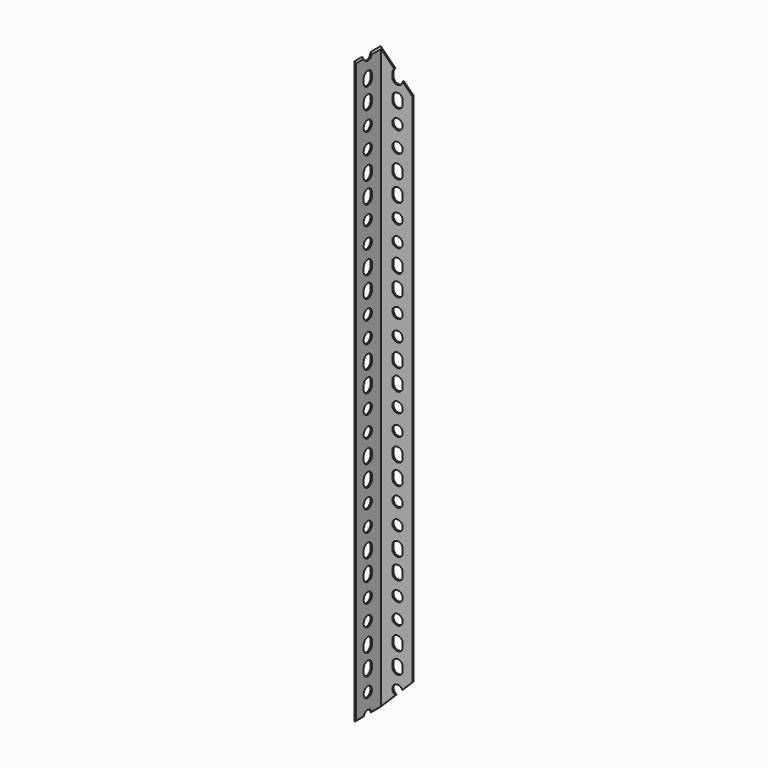
from build123d import *

# Parameters (mm, degrees)
F2_DEPTH = 533.4
F3_R     = 4.7625
F5_DEPTH = 1.3726
F4_R     = 4.7625
F6_DEPTH = 1.3726
F8_DEPTH = 30.1254


# Not quite as in the source:
# - a variable given as a bare number and used for a length is read in inches; the dataset says mm whatever the document's units were


with BuildPart() as f2:
    # F1 (on Top) → F2 (new body)
    with BuildSketch(Plane.XY):
        Polygon((-1.3716, 1.3716), (-1.3716, -28.7528), (0, -28.7528), (0, 0), (28.7528, 0), (28.7528, 1.3716), align=None)
    extrude(amount=F2_DEPTH)

    # F3 (on face) → F5 (cut, through all)
    with BuildSketch(Plane.XZ):
        with Locations((15.1384, 19.05)):
            Circle(F3_R)
        with Locations((15.1384, 0)):
            Circle(F3_R)
        with BuildLine():
            Line((19.9009, 36.5125), (19.9009, 39.6875))
            ThreePointArc((19.9009, 39.6875), (15.1384, 44.45), (10.3759, 39.6875))
            Line((10.3759, 39.6875), (10.3759, 36.5125))
            ThreePointArc((10.3759, 36.5125), (15.1384, 31.75), (19.9009, 36.5125))
        make_face()
        with BuildLine():
            Line((19.9009, 55.5625), (19.9009, 58.7375))
            ThreePointArc((19.9009, 58.7375), (15.1384, 63.5), (10.3759, 58.7375))
            Line((10.3759, 58.7375), (10.3759, 55.5625))
            ThreePointArc((10.3759, 55.5625), (15.1384, 50.8), (19.9009, 55.5625))
        make_face()
        with BuildLine():
            Line((19.9009, 131.7625), (19.9009, 134.9375))
            ThreePointArc((19.9009, 134.9375), (15.1384, 139.7), (10.3759, 134.9375))
            Line((10.3759, 134.9375), (10.3759, 131.7625))
            ThreePointArc((10.3759, 131.7625), (15.1384, 127), (19.9009, 131.7625))
        make_face()
        with Locations((15.1384, 95.25)):
            Circle(F3_R)
        with Locations((15.1384, 76.2)):
            Circle(F3_R)
        with BuildLine():
            Line((19.9009, 112.7125), (19.9009, 115.8875))
            ThreePointArc((19.9009, 115.8875), (15.1384, 120.65), (10.3759, 115.8875))
            Line((10.3759, 115.8875), (10.3759, 112.7125))
            ThreePointArc((10.3759, 112.7125), (15.1384, 107.95), (19.9009, 112.7125))
        make_face()
        with BuildLine():
            Line((19.9009, 207.9625), (19.9009, 211.1375))
            ThreePointArc((19.9009, 211.1375), (15.1384, 215.9), (10.3759, 211.1375))
            Line((10.3759, 211.1375), (10.3759, 207.9625))
            ThreePointArc((10.3759, 207.9625), (15.1384, 203.2), (19.9009, 207.9625))
        make_face()
        with Locations((15.1384, 171.45)):
            Circle(F3_R)
        with Locations((15.1384, 152.4)):
            Circle(F3_R)
        with BuildLine():
            Line((19.9009, 188.9125), (19.9009, 192.0875))
            ThreePointArc((19.9009, 192.0875), (15.1384, 196.85), (10.3759, 192.0875))
            Line((10.3759, 192.0875), (10.3759, 188.9125))
            ThreePointArc((10.3759, 188.9125), (15.1384, 184.15), (19.9009, 188.9125))
        make_face()
        with BuildLine():
            Line((19.9009, 284.1625), (19.9009, 287.3375))
            ThreePointArc((19.9009, 287.3375), (15.1384, 292.1), (10.3759, 287.3375))
            Line((10.3759, 287.3375), (10.3759, 284.1625))
            ThreePointArc((10.3759, 284.1625), (15.1384, 279.4), (19.9009, 284.1625))
        make_face()
        with Locations((15.1384, 247.65)):
            Circle(F3_R)
        with Locations((15.1384, 228.6)):
            Circle(F3_R)
        with BuildLine():
            Line((19.9009, 265.1125), (19.9009, 268.2875))
            ThreePointArc((19.9009, 268.2875), (15.1384, 273.05), (10.3759, 268.2875))
            Line((10.3759, 268.2875), (10.3759, 265.1125))
            ThreePointArc((10.3759, 265.1125), (15.1384, 260.35), (19.9009, 265.1125))
        make_face()
        with BuildLine():
            Line((19.9009, 360.3625), (19.9009, 363.5375))
            ThreePointArc((19.9009, 363.5375), (15.1384, 368.3), (10.3759, 363.5375))
            Line((10.3759, 363.5375), (10.3759, 360.3625))
            ThreePointArc((10.3759, 360.3625), (15.1384, 355.6), (19.9009, 360.3625))
        make_face()
        with Locations((15.1384, 323.85)):
            Circle(F3_R)
        with Locations((15.1384, 304.8)):
            Circle(F3_R)
        with BuildLine():
            Line((19.9009, 341.3125), (19.9009, 344.4875))
            ThreePointArc((19.9009, 344.4875), (15.1384, 349.25), (10.3759, 344.4875))
            Line((10.3759, 344.4875), (10.3759, 341.3125))
            ThreePointArc((10.3759, 341.3125), (15.1384, 336.55), (19.9009, 341.3125))
        make_face()
        with BuildLine():
            Line((19.9009, 436.5625), (19.9009, 439.7375))
            ThreePointArc((19.9009, 439.7375), (15.1384, 444.5), (10.3759, 439.7375))
            Line((10.3759, 439.7375), (10.3759, 436.5625))
            ThreePointArc((10.3759, 436.5625), (15.1384, 431.8), (19.9009, 436.5625))
        make_face()
        with Locations((15.1384, 400.05)):
            Circle(F3_R)
        with Locations((15.1384, 381)):
            Circle(F3_R)
        with BuildLine():
            Line((19.9009, 417.5125), (19.9009, 420.6875))
            ThreePointArc((19.9009, 420.6875), (15.1384, 425.45), (10.3759, 420.6875))
            Line((10.3759, 420.6875), (10.3759, 417.5125))
            ThreePointArc((10.3759, 417.5125), (15.1384, 412.75), (19.9009, 417.5125))
        make_face()
        with BuildLine():
            Line((19.9009, 512.7625), (19.9009, 515.9375))
            ThreePointArc((19.9009, 515.9375), (15.1384, 520.7), (10.3759, 515.9375))
            Line((10.3759, 515.9375), (10.3759, 512.7625))
            ThreePointArc((10.3759, 512.7625), (15.1384, 508), (19.9009, 512.7625))
        make_face()
        with Locations((15.1384, 476.25)):
            Circle(F3_R)
        with Locations((15.1384, 457.2)):
            Circle(F3_R)
        with BuildLine():
            Line((19.9009, 493.7125), (19.9009, 496.8875))
            ThreePointArc((19.9009, 496.8875), (15.1384, 501.65), (10.3759, 496.8875))
            Line((10.3759, 496.8875), (10.3759, 493.7125))
            ThreePointArc((10.3759, 493.7125), (15.1384, 488.95), (19.9009, 493.7125))
        make_face()
        with BuildLine():
            Line((19.9009, 588.9625), (19.9009, 592.1375))
            ThreePointArc((19.9009, 592.1375), (15.1384, 596.9), (10.3759, 592.1375))
            Line((10.3759, 592.1375), (10.3759, 588.9625))
            ThreePointArc((10.3759, 588.9625), (15.1384, 584.2), (19.9009, 588.9625))
        make_face()
        with Locations((15.1384, 552.45)):
            Circle(F3_R)
        with Locations((15.1384, 533.4)):
            Circle(F3_R)
        with BuildLine():
            Line((19.9009, 569.9125), (19.9009, 573.0875))
            ThreePointArc((19.9009, 573.0875), (15.1384, 577.85), (10.3759, 573.0875))
            Line((10.3759, 573.0875), (10.3759, 569.9125))
            ThreePointArc((10.3759, 569.9125), (15.1384, 565.15), (19.9009, 569.9125))
        make_face()
        with BuildLine():
            Line((19.9009, 665.1625), (19.9009, 668.3375))
            ThreePointArc((19.9009, 668.3375), (15.1384, 673.1), (10.3759, 668.3375))
            Line((10.3759, 668.3375), (10.3759, 665.1625))
            ThreePointArc((10.3759, 665.1625), (15.1384, 660.4), (19.9009, 665.1625))
        make_face()
        with Locations((15.1384, 628.65)):
            Circle(F3_R)
        with Locations((15.1384, 609.6)):
            Circle(F3_R)
        with BuildLine():
            Line((19.9009, 646.1125), (19.9009, 649.2875))
            ThreePointArc((19.9009, 649.2875), (15.1384, 654.05), (10.3759, 649.2875))
            Line((10.3759, 649.2875), (10.3759, 646.1125))
            ThreePointArc((10.3759, 646.1125), (15.1384, 641.35), (19.9009, 646.1125))
        make_face()
        with BuildLine():
            Line((19.9009, 741.3625), (19.9009, 744.5375))
            ThreePointArc((19.9009, 744.5375), (15.1384, 749.3), (10.3759, 744.5375))
            Line((10.3759, 744.5375), (10.3759, 741.3625))
            ThreePointArc((10.3759, 741.3625), (15.1384, 736.6), (19.9009, 741.3625))
        make_face()
        with Locations((15.1384, 704.85)):
            Circle(F3_R)
        with Locations((15.1384, 685.8)):
            Circle(F3_R)
        with BuildLine():
            Line((19.9009, 722.3125), (19.9009, 725.4875))
            ThreePointArc((19.9009, 725.4875), (15.1384, 730.25), (10.3759, 725.4875))
            Line((10.3759, 725.4875), (10.3759, 722.3125))
            ThreePointArc((10.3759, 722.3125), (15.1384, 717.55), (19.9009, 722.3125))
        make_face()
        with BuildLine():
            Line((19.9009, 817.5625), (19.9009, 820.7375))
            ThreePointArc((19.9009, 820.7375), (15.1384, 825.5), (10.3759, 820.7375))
            Line((10.3759, 820.7375), (10.3759, 817.5625))
            ThreePointArc((10.3759, 817.5625), (15.1384, 812.8), (19.9009, 817.5625))
        make_face()
        with Locations((15.1384, 781.05)):
            Circle(F3_R)
        with Locations((15.1384, 762)):
            Circle(F3_R)
        with BuildLine():
            Line((19.9009, 798.5125), (19.9009, 801.6875))
            ThreePointArc((19.9009, 801.6875), (15.1384, 806.45), (10.3759, 801.6875))
            Line((10.3759, 801.6875), (10.3759, 798.5125))
            ThreePointArc((10.3759, 798.5125), (15.1384, 793.75), (19.9009, 798.5125))
        make_face()
        with BuildLine():
            Line((19.9009, 893.7625), (19.9009, 896.9375))
            ThreePointArc((19.9009, 896.9375), (15.1384, 901.7), (10.3759, 896.9375))
            Line((10.3759, 896.9375), (10.3759, 893.7625))
            ThreePointArc((10.3759, 893.7625), (15.1384, 889), (19.9009, 893.7625))
        make_face()
        with Locations((15.1384, 857.25)):
            Circle(F3_R)
        with Locations((15.1384, 838.2)):
            Circle(F3_R)
        with BuildLine():
            Line((19.9009, 874.7125), (19.9009, 877.8875))
            ThreePointArc((19.9009, 877.8875), (15.1384, 882.65), (10.3759, 877.8875))
            Line((10.3759, 877.8875), (10.3759, 874.7125))
            ThreePointArc((10.3759, 874.7125), (15.1384, 869.95), (19.9009, 874.7125))
        make_face()
        with BuildLine():
            Line((19.9009, 969.9625), (19.9009, 973.1375))
            ThreePointArc((19.9009, 973.1375), (15.1384, 977.9), (10.3759, 973.1375))
            Line((10.3759, 973.1375), (10.3759, 969.9625))
            ThreePointArc((10.3759, 969.9625), (15.1384, 965.2), (19.9009, 969.9625))
        make_face()
        with Locations((15.1384, 933.45)):
            Circle(F3_R)
        with Locations((15.1384, 914.4)):
            Circle(F3_R)
        with BuildLine():
            Line((19.9009, 950.9125), (19.9009, 954.0875))
            ThreePointArc((19.9009, 954.0875), (15.1384, 958.85), (10.3759, 954.0875))
            Line((10.3759, 954.0875), (10.3759, 950.9125))
            ThreePointArc((10.3759, 950.9125), (15.1384, 946.15), (19.9009, 950.9125))
        make_face()
        with BuildLine():
            Line((19.9009, 1046.1625), (19.9009, 1049.3375))
            ThreePointArc((19.9009, 1049.3375), (15.1384, 1054.1), (10.3759, 1049.3375))
            Line((10.3759, 1049.3375), (10.3759, 1046.1625))
            ThreePointArc((10.3759, 1046.1625), (15.1384, 1041.4), (19.9009, 1046.1625))
        make_face()
        with Locations((15.1384, 1009.65)):
            Circle(F3_R)
        with Locations((15.1384, 990.6)):
            Circle(F3_R)
        with BuildLine():
            Line((19.9009, 1027.1125), (19.9009, 1030.2875))
            ThreePointArc((19.9009, 1030.2875), (15.1384, 1035.05), (10.3759, 1030.2875))
            Line((10.3759, 1030.2875), (10.3759, 1027.1125))
            ThreePointArc((10.3759, 1027.1125), (15.1384, 1022.35), (19.9009, 1027.1125))
        make_face()
        with BuildLine():
            Line((19.9009, 1122.3625), (19.9009, 1125.5375))
            ThreePointArc((19.9009, 1125.5375), (15.1384, 1130.3), (10.3759, 1125.5375))
            Line((10.3759, 1125.5375), (10.3759, 1122.3625))
            ThreePointArc((10.3759, 1122.3625), (15.1384, 1117.6), (19.9009, 1122.3625))
        make_face()
        with Locations((15.1384, 1085.85)):
            Circle(F3_R)
        with Locations((15.1384, 1066.8)):
            Circle(F3_R)
        with BuildLine():
            Line((19.9009, 1103.3125), (19.9009, 1106.4875))
            ThreePointArc((19.9009, 1106.4875), (15.1384, 1111.25), (10.3759, 1106.4875))
            Line((10.3759, 1106.4875), (10.3759, 1103.3125))
            ThreePointArc((10.3759, 1103.3125), (15.1384, 1098.55), (19.9009, 1103.3125))
        make_face()
        with BuildLine():
            Line((19.9009, 1198.5625), (19.9009, 1201.7375))
            ThreePointArc((19.9009, 1201.7375), (15.1384, 1206.5), (10.3759, 1201.7375))
            Line((10.3759, 1201.7375), (10.3759, 1198.5625))
            ThreePointArc((10.3759, 1198.5625), (15.1384, 1193.8), (19.9009, 1198.5625))
        make_face()
        with Locations((15.1384, 1162.05)):
            Circle(F3_R)
        with Locations((15.1384, 1143)):
            Circle(F3_R)
        with BuildLine():
            Line((19.9009, 1179.5125), (19.9009, 1182.6875))
            ThreePointArc((19.9009, 1182.6875), (15.1384, 1187.45), (10.3759, 1182.6875))
            Line((10.3759, 1182.6875), (10.3759, 1179.5125))
            ThreePointArc((10.3759, 1179.5125), (15.1384, 1174.75), (19.9009, 1179.5125))
        make_face()
        with BuildLine():
            Line((19.9009, 1274.7625), (19.9009, 1277.9375))
            ThreePointArc((19.9009, 1277.9375), (15.1384, 1282.7), (10.3759, 1277.9375))
            Line((10.3759, 1277.9375), (10.3759, 1274.7625))
            ThreePointArc((10.3759, 1274.7625), (15.1384, 1270), (19.9009, 1274.7625))
        make_face()
        with Locations((15.1384, 1238.25)):
            Circle(F3_R)
        with Locations((15.1384, 1219.2)):
            Circle(F3_R)
        with BuildLine():
            Line((19.9009, 1255.7125), (19.9009, 1258.8875))
            ThreePointArc((19.9009, 1258.8875), (15.1384, 1263.65), (10.3759, 1258.8875))
            Line((10.3759, 1258.8875), (10.3759, 1255.7125))
            ThreePointArc((10.3759, 1255.7125), (15.1384, 1250.95), (19.9009, 1255.7125))
        make_face()
        with BuildLine():
            Line((19.9009, 1350.9625), (19.9009, 1354.1375))
            ThreePointArc((19.9009, 1354.1375), (15.1384, 1358.9), (10.3759, 1354.1375))
            Line((10.3759, 1354.1375), (10.3759, 1350.9625))
            ThreePointArc((10.3759, 1350.9625), (15.1384, 1346.2), (19.9009, 1350.9625))
        make_face()
        with Locations((15.1384, 1314.45)):
            Circle(F3_R)
        with Locations((15.1384, 1295.4)):
            Circle(F3_R)
        with BuildLine():
            Line((19.9009, 1331.9125), (19.9009, 1335.0875))
            ThreePointArc((19.9009, 1335.0875), (15.1384, 1339.85), (10.3759, 1335.0875))
            Line((10.3759, 1335.0875), (10.3759, 1331.9125))
            ThreePointArc((10.3759, 1331.9125), (15.1384, 1327.15), (19.9009, 1331.9125))
        make_face()
        with BuildLine():
            Line((19.9009, 1427.1625), (19.9009, 1430.3375))
            ThreePointArc((19.9009, 1430.3375), (15.1384, 1435.1), (10.3759, 1430.3375))
            Line((10.3759, 1430.3375), (10.3759, 1427.1625))
            ThreePointArc((10.3759, 1427.1625), (15.1384, 1422.4), (19.9009, 1427.1625))
        make_face()
        with Locations((15.1384, 1390.65)):
            Circle(F3_R)
        with Locations((15.1384, 1371.6)):
            Circle(F3_R)
        with BuildLine():
            Line((19.9009, 1408.1125), (19.9009, 1411.2875))
            ThreePointArc((19.9009, 1411.2875), (15.1384, 1416.05), (10.3759, 1411.2875))
            Line((10.3759, 1411.2875), (10.3759, 1408.1125))
            ThreePointArc((10.3759, 1408.1125), (15.1384, 1403.35), (19.9009, 1408.1125))
        make_face()
        with BuildLine():
            Line((19.9009, 1503.3625), (19.9009, 1506.5375))
            ThreePointArc((19.9009, 1506.5375), (15.1384, 1511.3), (10.3759, 1506.5375))
            Line((10.3759, 1506.5375), (10.3759, 1503.3625))
            ThreePointArc((10.3759, 1503.3625), (15.1384, 1498.6), (19.9009, 1503.3625))
        make_face()
        with Locations((15.1384, 1466.85)):
            Circle(F3_R)
        with Locations((15.1384, 1447.8)):
            Circle(F3_R)
        with BuildLine():
            Line((19.9009, 1484.3125), (19.9009, 1487.4875))
            ThreePointArc((19.9009, 1487.4875), (15.1384, 1492.25), (10.3759, 1487.4875))
            Line((10.3759, 1487.4875), (10.3759, 1484.3125))
            ThreePointArc((10.3759, 1484.3125), (15.1384, 1479.55), (19.9009, 1484.3125))
        make_face()
        with BuildLine():
            Line((19.9009, 1579.5625), (19.9009, 1582.7375))
            ThreePointArc((19.9009, 1582.7375), (15.1384, 1587.5), (10.3759, 1582.7375))
            Line((10.3759, 1582.7375), (10.3759, 1579.5625))
            ThreePointArc((10.3759, 1579.5625), (15.1384, 1574.8), (19.9009, 1579.5625))
        make_face()
        with Locations((15.1384, 1543.05)):
            Circle(F3_R)
        with Locations((15.1384, 1524)):
            Circle(F3_R)
        with BuildLine():
            Line((19.9009, 1560.5125), (19.9009, 1563.6875))
            ThreePointArc((19.9009, 1563.6875), (15.1384, 1568.45), (10.3759, 1563.6875))
            Line((10.3759, 1563.6875), (10.3759, 1560.5125))
            ThreePointArc((10.3759, 1560.5125), (15.1384, 1555.75), (19.9009, 1560.5125))
        make_face()
        with BuildLine():
            Line((19.9009, 1655.7625), (19.9009, 1658.9375))
            ThreePointArc((19.9009, 1658.9375), (15.1384, 1663.7), (10.3759, 1658.9375))
            Line((10.3759, 1658.9375), (10.3759, 1655.7625))
            ThreePointArc((10.3759, 1655.7625), (15.1384, 1651), (19.9009, 1655.7625))
        make_face()
        with Locations((15.1384, 1619.25)):
            Circle(F3_R)
        with Locations((15.1384, 1600.2)):
            Circle(F3_R)
        with BuildLine():
            Line((19.9009, 1636.7125), (19.9009, 1639.8875))
            ThreePointArc((19.9009, 1639.8875), (15.1384, 1644.65), (10.3759, 1639.8875))
            Line((10.3759, 1639.8875), (10.3759, 1636.7125))
            ThreePointArc((10.3759, 1636.7125), (15.1384, 1631.95), (19.9009, 1636.7125))
        make_face()
        with BuildLine():
            Line((19.9009, 1731.9625), (19.9009, 1735.1375))
            ThreePointArc((19.9009, 1735.1375), (15.1384, 1739.9), (10.3759, 1735.1375))
            Line((10.3759, 1735.1375), (10.3759, 1731.9625))
            ThreePointArc((10.3759, 1731.9625), (15.1384, 1727.2), (19.9009, 1731.9625))
        make_face()
        with Locations((15.1384, 1695.45)):
            Circle(F3_R)
        with Locations((15.1384, 1676.4)):
            Circle(F3_R)
        with BuildLine():
            Line((19.9009, 1712.9125), (19.9009, 1716.0875))
            ThreePointArc((19.9009, 1716.0875), (15.1384, 1720.85), (10.3759, 1716.0875))
            Line((10.3759, 1716.0875), (10.3759, 1712.9125))
            ThreePointArc((10.3759, 1712.9125), (15.1384, 1708.15), (19.9009, 1712.9125))
        make_face()
        with BuildLine():
            Line((19.9009, 1808.1625), (19.9009, 1811.3375))
            ThreePointArc((19.9009, 1811.3375), (15.1384, 1816.1), (10.3759, 1811.3375))
            Line((10.3759, 1811.3375), (10.3759, 1808.1625))
            ThreePointArc((10.3759, 1808.1625), (15.1384, 1803.4), (19.9009, 1808.1625))
        make_face()
        with Locations((15.1384, 1771.65)):
            Circle(F3_R)
        with Locations((15.1384, 1752.6)):
            Circle(F3_R)
        with BuildLine():
            Line((19.9009, 1789.1125), (19.9009, 1792.2875))
            ThreePointArc((19.9009, 1792.2875), (15.1384, 1797.05), (10.3759, 1792.2875))
            Line((10.3759, 1792.2875), (10.3759, 1789.1125))
            ThreePointArc((10.3759, 1789.1125), (15.1384, 1784.35), (19.9009, 1789.1125))
        make_face()
    extrude(amount=-F5_DEPTH, mode=Mode.SUBTRACT)

    # F4 (on face) → F6 (cut, through all)
    with BuildSketch(Plane.YZ):
        with Locations((-15.1384, 19.05)):
            Circle(F4_R)
        with Locations((-15.1384, 0)):
            Circle(F4_R)
        with BuildLine():
            Line((-10.3759, 36.5125), (-10.3759, 39.6875))
            ThreePointArc((-10.3759, 39.6875), (-15.1384, 44.45), (-19.9009, 39.6875))
            Line((-19.9009, 39.6875), (-19.9009, 36.5125))
            ThreePointArc((-19.9009, 36.5125), (-15.1384, 31.75), (-10.3759, 36.5125))
        make_face()
        with BuildLine():
            Line((-10.3759, 55.5625), (-10.3759, 58.7375))
            ThreePointArc((-10.3759, 58.7375), (-15.1384, 63.5), (-19.9009, 58.7375))
            Line((-19.9009, 58.7375), (-19.9009, 55.5625))
            ThreePointArc((-19.9009, 55.5625), (-15.1384, 50.8), (-10.3759, 55.5625))
        make_face()
        with BuildLine():
            Line((-10.3759, 131.7625), (-10.3759, 134.9375))
            ThreePointArc((-10.3759, 134.9375), (-15.1384, 139.7), (-19.9009, 134.9375))
            Line((-19.9009, 134.9375), (-19.9009, 131.7625))
            ThreePointArc((-19.9009, 131.7625), (-15.1384, 127), (-10.3759, 131.7625))
        make_face()
        with Locations((-15.1384, 95.25)):
            Circle(F4_R)
        with Locations((-15.1384, 76.2)):
            Circle(F4_R)
        with BuildLine():
            Line((-10.3759, 112.7125), (-10.3759, 115.8875))
            ThreePointArc((-10.3759, 115.8875), (-15.1384, 120.65), (-19.9009, 115.8875))
            Line((-19.9009, 115.8875), (-19.9009, 112.7125))
            ThreePointArc((-19.9009, 112.7125), (-15.1384, 107.95), (-10.3759, 112.7125))
        make_face()
        with BuildLine():
            Line((-10.3759, 207.9625), (-10.3759, 211.1375))
            ThreePointArc((-10.3759, 211.1375), (-15.1384, 215.9), (-19.9009, 211.1375))
            Line((-19.9009, 211.1375), (-19.9009, 207.9625))
            ThreePointArc((-19.9009, 207.9625), (-15.1384, 203.2), (-10.3759, 207.9625))
        make_face()
        with Locations((-15.1384, 171.45)):
            Circle(F4_R)
        with Locations((-15.1384, 152.4)):
            Circle(F4_R)
        with BuildLine():
            Line((-10.3759, 188.9125), (-10.3759, 192.0875))
            ThreePointArc((-10.3759, 192.0875), (-15.1384, 196.85), (-19.9009, 192.0875))
            Line((-19.9009, 192.0875), (-19.9009, 188.9125))
            ThreePointArc((-19.9009, 188.9125), (-15.1384, 184.15), (-10.3759, 188.9125))
        make_face()
        with BuildLine():
            Line((-10.3759, 284.1625), (-10.3759, 287.3375))
            ThreePointArc((-10.3759, 287.3375), (-15.1384, 292.1), (-19.9009, 287.3375))
            Line((-19.9009, 287.3375), (-19.9009, 284.1625))
            ThreePointArc((-19.9009, 284.1625), (-15.1384, 279.4), (-10.3759, 284.1625))
        make_face()
        with Locations((-15.1384, 247.65)):
            Circle(F4_R)
        with Locations((-15.1384, 228.6)):
            Circle(F4_R)
        with BuildLine():
            Line((-10.3759, 265.1125), (-10.3759, 268.2875))
            ThreePointArc((-10.3759, 268.2875), (-15.1384, 273.05), (-19.9009, 268.2875))
            Line((-19.9009, 268.2875), (-19.9009, 265.1125))
            ThreePointArc((-19.9009, 265.1125), (-15.1384, 260.35), (-10.3759, 265.1125))
        make_face()
        with BuildLine():
            Line((-10.3759, 360.3625), (-10.3759, 363.5375))
            ThreePointArc((-10.3759, 363.5375), (-15.1384, 368.3), (-19.9009, 363.5375))
            Line((-19.9009, 363.5375), (-19.9009, 360.3625))
            ThreePointArc((-19.9009, 360.3625), (-15.1384, 355.6), (-10.3759, 360.3625))
        make_face()
        with Locations((-15.1384, 323.85)):
            Circle(F4_R)
        with Locations((-15.1384, 304.8)):
            Circle(F4_R)
        with BuildLine():
            Line((-10.3759, 341.3125), (-10.3759, 344.4875))
            ThreePointArc((-10.3759, 344.4875), (-15.1384, 349.25), (-19.9009, 344.4875))
            Line((-19.9009, 344.4875), (-19.9009, 341.3125))
            ThreePointArc((-19.9009, 341.3125), (-15.1384, 336.55), (-10.3759, 341.3125))
        make_face()
        with BuildLine():
            Line((-10.3759, 436.5625), (-10.3759, 439.7375))
            ThreePointArc((-10.3759, 439.7375), (-15.1384, 444.5), (-19.9009, 439.7375))
            Line((-19.9009, 439.7375), (-19.9009, 436.5625))
            ThreePointArc((-19.9009, 436.5625), (-15.1384, 431.8), (-10.3759, 436.5625))
        make_face()
        with Locations((-15.1384, 400.05)):
            Circle(F4_R)
        with Locations((-15.1384, 381)):
            Circle(F4_R)
        with BuildLine():
            Line((-10.3759, 417.5125), (-10.3759, 420.6875))
            ThreePointArc((-10.3759, 420.6875), (-15.1384, 425.45), (-19.9009, 420.6875))
            Line((-19.9009, 420.6875), (-19.9009, 417.5125))
            ThreePointArc((-19.9009, 417.5125), (-15.1384, 412.75), (-10.3759, 417.5125))
        make_face()
        with BuildLine():
            Line((-10.3759, 512.7625), (-10.3759, 515.9375))
            ThreePointArc((-10.3759, 515.9375), (-15.1384, 520.7), (-19.9009, 515.9375))
            Line((-19.9009, 515.9375), (-19.9009, 512.7625))
            ThreePointArc((-19.9009, 512.7625), (-15.1384, 508), (-10.3759, 512.7625))
        make_face()
        with Locations((-15.1384, 476.25)):
            Circle(F4_R)
        with Locations((-15.1384, 457.2)):
            Circle(F4_R)
        with BuildLine():
            Line((-10.3759, 493.7125), (-10.3759, 496.8875))
            ThreePointArc((-10.3759, 496.8875), (-15.1384, 501.65), (-19.9009, 496.8875))
            Line((-19.9009, 496.8875), (-19.9009, 493.7125))
            ThreePointArc((-19.9009, 493.7125), (-15.1384, 488.95), (-10.3759, 493.7125))
        make_face()
        with BuildLine():
            Line((-10.3759, 588.9625), (-10.3759, 592.1375))
            ThreePointArc((-10.3759, 592.1375), (-15.1384, 596.9), (-19.9009, 592.1375))
            Line((-19.9009, 592.1375), (-19.9009, 588.9625))
            ThreePointArc((-19.9009, 588.9625), (-15.1384, 584.2), (-10.3759, 588.9625))
        make_face()
        with Locations((-15.1384, 552.45)):
            Circle(F4_R)
        with Locations((-15.1384, 533.4)):
            Circle(F4_R)
        with BuildLine():
            Line((-10.3759, 569.9125), (-10.3759, 573.0875))
            ThreePointArc((-10.3759, 573.0875), (-15.1384, 577.85), (-19.9009, 573.0875))
            Line((-19.9009, 573.0875), (-19.9009, 569.9125))
            ThreePointArc((-19.9009, 569.9125), (-15.1384, 565.15), (-10.3759, 569.9125))
        make_face()
        with BuildLine():
            Line((-10.3759, 665.1625), (-10.3759, 668.3375))
            ThreePointArc((-10.3759, 668.3375), (-15.1384, 673.1), (-19.9009, 668.3375))
            Line((-19.9009, 668.3375), (-19.9009, 665.1625))
            ThreePointArc((-19.9009, 665.1625), (-15.1384, 660.4), (-10.3759, 665.1625))
        make_face()
        with Locations((-15.1384, 628.65)):
            Circle(F4_R)
        with Locations((-15.1384, 609.6)):
            Circle(F4_R)
        with BuildLine():
            Line((-10.3759, 646.1125), (-10.3759, 649.2875))
            ThreePointArc((-10.3759, 649.2875), (-15.1384, 654.05), (-19.9009, 649.2875))
            Line((-19.9009, 649.2875), (-19.9009, 646.1125))
            ThreePointArc((-19.9009, 646.1125), (-15.1384, 641.35), (-10.3759, 646.1125))
        make_face()
        with BuildLine():
            Line((-10.3759, 741.3625), (-10.3759, 744.5375))
            ThreePointArc((-10.3759, 744.5375), (-15.1384, 749.3), (-19.9009, 744.5375))
            Line((-19.9009, 744.5375), (-19.9009, 741.3625))
            ThreePointArc((-19.9009, 741.3625), (-15.1384, 736.6), (-10.3759, 741.3625))
        make_face()
        with Locations((-15.1384, 704.85)):
            Circle(F4_R)
        with Locations((-15.1384, 685.8)):
            Circle(F4_R)
        with BuildLine():
            Line((-10.3759, 722.3125), (-10.3759, 725.4875))
            ThreePointArc((-10.3759, 725.4875), (-15.1384, 730.25), (-19.9009, 725.4875))
            Line((-19.9009, 725.4875), (-19.9009, 722.3125))
            ThreePointArc((-19.9009, 722.3125), (-15.1384, 717.55), (-10.3759, 722.3125))
        make_face()
        with BuildLine():
            Line((-10.3759, 817.5625), (-10.3759, 820.7375))
            ThreePointArc((-10.3759, 820.7375), (-15.1384, 825.5), (-19.9009, 820.7375))
            Line((-19.9009, 820.7375), (-19.9009, 817.5625))
            ThreePointArc((-19.9009, 817.5625), (-15.1384, 812.8), (-10.3759, 817.5625))
        make_face()
        with Locations((-15.1384, 781.05)):
            Circle(F4_R)
        with Locations((-15.1384, 762)):
            Circle(F4_R)
        with BuildLine():
            Line((-10.3759, 798.5125), (-10.3759, 801.6875))
            ThreePointArc((-10.3759, 801.6875), (-15.1384, 806.45), (-19.9009, 801.6875))
            Line((-19.9009, 801.6875), (-19.9009, 798.5125))
            ThreePointArc((-19.9009, 798.5125), (-15.1384, 793.75), (-10.3759, 798.5125))
        make_face()
        with BuildLine():
            Line((-10.3759, 893.7625), (-10.3759, 896.9375))
            ThreePointArc((-10.3759, 896.9375), (-15.1384, 901.7), (-19.9009, 896.9375))
            Line((-19.9009, 896.9375), (-19.9009, 893.7625))
            ThreePointArc((-19.9009, 893.7625), (-15.1384, 889), (-10.3759, 893.7625))
        make_face()
        with Locations((-15.1384, 857.25)):
            Circle(F4_R)
        with Locations((-15.1384, 838.2)):
            Circle(F4_R)
        with BuildLine():
            Line((-10.3759, 874.7125), (-10.3759, 877.8875))
            ThreePointArc((-10.3759, 877.8875), (-15.1384, 882.65), (-19.9009, 877.8875))
            Line((-19.9009, 877.8875), (-19.9009, 874.7125))
            ThreePointArc((-19.9009, 874.7125), (-15.1384, 869.95), (-10.3759, 874.7125))
        make_face()
        with BuildLine():
            Line((-10.3759, 969.9625), (-10.3759, 973.1375))
            ThreePointArc((-10.3759, 973.1375), (-15.1384, 977.9), (-19.9009, 973.1375))
            Line((-19.9009, 973.1375), (-19.9009, 969.9625))
            ThreePointArc((-19.9009, 969.9625), (-15.1384, 965.2), (-10.3759, 969.9625))
        make_face()
        with Locations((-15.1384, 933.45)):
            Circle(F4_R)
        with Locations((-15.1384, 914.4)):
            Circle(F4_R)
        with BuildLine():
            Line((-10.3759, 950.9125), (-10.3759, 954.0875))
            ThreePointArc((-10.3759, 954.0875), (-15.1384, 958.85), (-19.9009, 954.0875))
            Line((-19.9009, 954.0875), (-19.9009, 950.9125))
            ThreePointArc((-19.9009, 950.9125), (-15.1384, 946.15), (-10.3759, 950.9125))
        make_face()
        with BuildLine():
            Line((-10.3759, 1046.1625), (-10.3759, 1049.3375))
            ThreePointArc((-10.3759, 1049.3375), (-15.1384, 1054.1), (-19.9009, 1049.3375))
            Line((-19.9009, 1049.3375), (-19.9009, 1046.1625))
            ThreePointArc((-19.9009, 1046.1625), (-15.1384, 1041.4), (-10.3759, 1046.1625))
        make_face()
        with Locations((-15.1384, 1009.65)):
            Circle(F4_R)
        with Locations((-15.1384, 990.6)):
            Circle(F4_R)
        with BuildLine():
            Line((-10.3759, 1027.1125), (-10.3759, 1030.2875))
            ThreePointArc((-10.3759, 1030.2875), (-15.1384, 1035.05), (-19.9009, 1030.2875))
            Line((-19.9009, 1030.2875), (-19.9009, 1027.1125))
            ThreePointArc((-19.9009, 1027.1125), (-15.1384, 1022.35), (-10.3759, 1027.1125))
        make_face()
        with BuildLine():
            Line((-10.3759, 1122.3625), (-10.3759, 1125.5375))
            ThreePointArc((-10.3759, 1125.5375), (-15.1384, 1130.3), (-19.9009, 1125.5375))
            Line((-19.9009, 1125.5375), (-19.9009, 1122.3625))
            ThreePointArc((-19.9009, 1122.3625), (-15.1384, 1117.6), (-10.3759, 1122.3625))
        make_face()
        with Locations((-15.1384, 1085.85)):
            Circle(F4_R)
        with Locations((-15.1384, 1066.8)):
            Circle(F4_R)
        with BuildLine():
            Line((-10.3759, 1103.3125), (-10.3759, 1106.4875))
            ThreePointArc((-10.3759, 1106.4875), (-15.1384, 1111.25), (-19.9009, 1106.4875))
            Line((-19.9009, 1106.4875), (-19.9009, 1103.3125))
            ThreePointArc((-19.9009, 1103.3125), (-15.1384, 1098.55), (-10.3759, 1103.3125))
        make_face()
        with BuildLine():
            Line((-10.3759, 1198.5625), (-10.3759, 1201.7375))
            ThreePointArc((-10.3759, 1201.7375), (-15.1384, 1206.5), (-19.9009, 1201.7375))
            Line((-19.9009, 1201.7375), (-19.9009, 1198.5625))
            ThreePointArc((-19.9009, 1198.5625), (-15.1384, 1193.8), (-10.3759, 1198.5625))
        make_face()
        with Locations((-15.1384, 1162.05)):
            Circle(F4_R)
        with Locations((-15.1384, 1143)):
            Circle(F4_R)
        with BuildLine():
            Line((-10.3759, 1179.5125), (-10.3759, 1182.6875))
            ThreePointArc((-10.3759, 1182.6875), (-15.1384, 1187.45), (-19.9009, 1182.6875))
            Line((-19.9009, 1182.6875), (-19.9009, 1179.5125))
            ThreePointArc((-19.9009, 1179.5125), (-15.1384, 1174.75), (-10.3759, 1179.5125))
        make_face()
        with BuildLine():
            Line((-10.3759, 1274.7625), (-10.3759, 1277.9375))
            ThreePointArc((-10.3759, 1277.9375), (-15.1384, 1282.7), (-19.9009, 1277.9375))
            Line((-19.9009, 1277.9375), (-19.9009, 1274.7625))
            ThreePointArc((-19.9009, 1274.7625), (-15.1384, 1270), (-10.3759, 1274.7625))
        make_face()
        with Locations((-15.1384, 1238.25)):
            Circle(F4_R)
        with Locations((-15.1384, 1219.2)):
            Circle(F4_R)
        with BuildLine():
            Line((-10.3759, 1255.7125), (-10.3759, 1258.8875))
            ThreePointArc((-10.3759, 1258.8875), (-15.1384, 1263.65), (-19.9009, 1258.8875))
            Line((-19.9009, 1258.8875), (-19.9009, 1255.7125))
            ThreePointArc((-19.9009, 1255.7125), (-15.1384, 1250.95), (-10.3759, 1255.7125))
        make_face()
        with BuildLine():
            Line((-10.3759, 1350.9625), (-10.3759, 1354.1375))
            ThreePointArc((-10.3759, 1354.1375), (-15.1384, 1358.9), (-19.9009, 1354.1375))
            Line((-19.9009, 1354.1375), (-19.9009, 1350.9625))
            ThreePointArc((-19.9009, 1350.9625), (-15.1384, 1346.2), (-10.3759, 1350.9625))
        make_face()
        with Locations((-15.1384, 1314.45)):
            Circle(F4_R)
        with Locations((-15.1384, 1295.4)):
            Circle(F4_R)
        with BuildLine():
            Line((-10.3759, 1331.9125), (-10.3759, 1335.0875))
            ThreePointArc((-10.3759, 1335.0875), (-15.1384, 1339.85), (-19.9009, 1335.0875))
            Line((-19.9009, 1335.0875), (-19.9009, 1331.9125))
            ThreePointArc((-19.9009, 1331.9125), (-15.1384, 1327.15), (-10.3759, 1331.9125))
        make_face()
        with BuildLine():
            Line((-10.3759, 1427.1625), (-10.3759, 1430.3375))
            ThreePointArc((-10.3759, 1430.3375), (-15.1384, 1435.1), (-19.9009, 1430.3375))
            Line((-19.9009, 1430.3375), (-19.9009, 1427.1625))
            ThreePointArc((-19.9009, 1427.1625), (-15.1384, 1422.4), (-10.3759, 1427.1625))
        make_face()
        with Locations((-15.1384, 1390.65)):
            Circle(F4_R)
        with Locations((-15.1384, 1371.6)):
            Circle(F4_R)
        with BuildLine():
            Line((-10.3759, 1408.1125), (-10.3759, 1411.2875))
            ThreePointArc((-10.3759, 1411.2875), (-15.1384, 1416.05), (-19.9009, 1411.2875))
            Line((-19.9009, 1411.2875), (-19.9009, 1408.1125))
            ThreePointArc((-19.9009, 1408.1125), (-15.1384, 1403.35), (-10.3759, 1408.1125))
        make_face()
        with BuildLine():
            Line((-10.3759, 1503.3625), (-10.3759, 1506.5375))
            ThreePointArc((-10.3759, 1506.5375), (-15.1384, 1511.3), (-19.9009, 1506.5375))
            Line((-19.9009, 1506.5375), (-19.9009, 1503.3625))
            ThreePointArc((-19.9009, 1503.3625), (-15.1384, 1498.6), (-10.3759, 1503.3625))
        make_face()
        with Locations((-15.1384, 1466.85)):
            Circle(F4_R)
        with Locations((-15.1384, 1447.8)):
            Circle(F4_R)
        with BuildLine():
            Line((-10.3759, 1484.3125), (-10.3759, 1487.4875))
            ThreePointArc((-10.3759, 1487.4875), (-15.1384, 1492.25), (-19.9009, 1487.4875))
            Line((-19.9009, 1487.4875), (-19.9009, 1484.3125))
            ThreePointArc((-19.9009, 1484.3125), (-15.1384, 1479.55), (-10.3759, 1484.3125))
        make_face()
        with BuildLine():
            Line((-10.3759, 1579.5625), (-10.3759, 1582.7375))
            ThreePointArc((-10.3759, 1582.7375), (-15.1384, 1587.5), (-19.9009, 1582.7375))
            Line((-19.9009, 1582.7375), (-19.9009, 1579.5625))
            ThreePointArc((-19.9009, 1579.5625), (-15.1384, 1574.8), (-10.3759, 1579.5625))
        make_face()
        with Locations((-15.1384, 1543.05)):
            Circle(F4_R)
        with Locations((-15.1384, 1524)):
            Circle(F4_R)
        with BuildLine():
            Line((-10.3759, 1560.5125), (-10.3759, 1563.6875))
            ThreePointArc((-10.3759, 1563.6875), (-15.1384, 1568.45), (-19.9009, 1563.6875))
            Line((-19.9009, 1563.6875), (-19.9009, 1560.5125))
            ThreePointArc((-19.9009, 1560.5125), (-15.1384, 1555.75), (-10.3759, 1560.5125))
        make_face()
        with BuildLine():
            Line((-10.3759, 1655.7625), (-10.3759, 1658.9375))
            ThreePointArc((-10.3759, 1658.9375), (-15.1384, 1663.7), (-19.9009, 1658.9375))
            Line((-19.9009, 1658.9375), (-19.9009, 1655.7625))
            ThreePointArc((-19.9009, 1655.7625), (-15.1384, 1651), (-10.3759, 1655.7625))
        make_face()
        with Locations((-15.1384, 1619.25)):
            Circle(F4_R)
        with Locations((-15.1384, 1600.2)):
            Circle(F4_R)
        with BuildLine():
            Line((-10.3759, 1636.7125), (-10.3759, 1639.8875))
            ThreePointArc((-10.3759, 1639.8875), (-15.1384, 1644.65), (-19.9009, 1639.8875))
            Line((-19.9009, 1639.8875), (-19.9009, 1636.7125))
            ThreePointArc((-19.9009, 1636.7125), (-15.1384, 1631.95), (-10.3759, 1636.7125))
        make_face()
        with BuildLine():
            Line((-10.3759, 1731.9625), (-10.3759, 1735.1375))
            ThreePointArc((-10.3759, 1735.1375), (-15.1384, 1739.9), (-19.9009, 1735.1375))
            Line((-19.9009, 1735.1375), (-19.9009, 1731.9625))
            ThreePointArc((-19.9009, 1731.9625), (-15.1384, 1727.2), (-10.3759, 1731.9625))
        make_face()
        with Locations((-15.1384, 1695.45)):
            Circle(F4_R)
        with Locations((-15.1384, 1676.4)):
            Circle(F4_R)
        with BuildLine():
            Line((-10.3759, 1712.9125), (-10.3759, 1716.0875))
            ThreePointArc((-10.3759, 1716.0875), (-15.1384, 1720.85), (-19.9009, 1716.0875))
            Line((-19.9009, 1716.0875), (-19.9009, 1712.9125))
            ThreePointArc((-19.9009, 1712.9125), (-15.1384, 1708.15), (-10.3759, 1712.9125))
        make_face()
        with BuildLine():
            Line((-10.3759, 1808.1625), (-10.3759, 1811.3375))
            ThreePointArc((-10.3759, 1811.3375), (-15.1384, 1816.1), (-19.9009, 1811.3375))
            Line((-19.9009, 1811.3375), (-19.9009, 1808.1625))
            ThreePointArc((-19.9009, 1808.1625), (-15.1384, 1803.4), (-10.3759, 1808.1625))
        make_face()
        with Locations((-15.1384, 1771.65)):
            Circle(F4_R)
        with Locations((-15.1384, 1752.6)):
            Circle(F4_R)
        with BuildLine():
            Line((-10.3759, 1789.1125), (-10.3759, 1792.2875))
            ThreePointArc((-10.3759, 1792.2875), (-15.1384, 1797.05), (-19.9009, 1792.2875))
            Line((-19.9009, 1792.2875), (-19.9009, 1789.1125))
            ThreePointArc((-19.9009, 1789.1125), (-15.1384, 1784.35), (-10.3759, 1789.1125))
        make_face()
    extrude(amount=-F6_DEPTH, mode=Mode.SUBTRACT)

    # F7 (on face) → F8 (cut, through all)
    with BuildSketch(Plane(origin=(0, 1.3716, 0), x_dir=(-1, 0, 0), z_dir=(0, 1, 0))):
        Polygon((-28.7528, 503.2756), (1.3716, 533.4), (-28.7528, 533.4), align=None)
        Polygon((-28.7528, 30.1244), (-28.7528, 0), (1.3716, 0), align=None)
    extrude(amount=-F8_DEPTH, mode=Mode.SUBTRACT)


solid = f2.part
